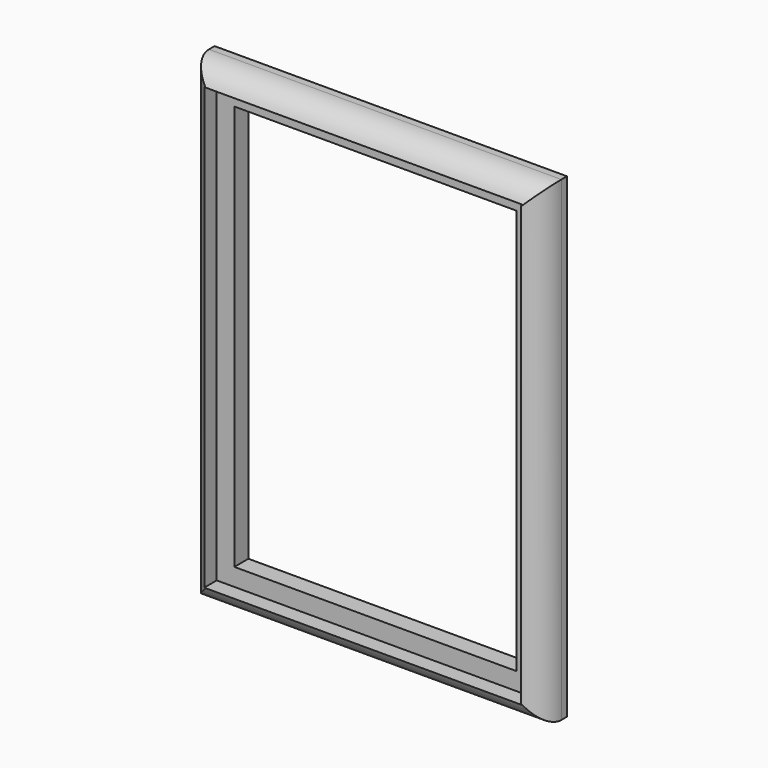
from build123d import *

# Parameters (mm, degrees)
F0_W        = 200
F0_H        = 270
F1_DEPTH    = 20
F2_W        = 180
F2_H        = 250
F3_DEPTH    = 10
F4_W        = 160
F4_H        = 230
F5_DEPTH    = 25
F6_T1_DEPTH = 350
F6_T3_DEPTH = 280


# Not quite as in the source:
# - a fillet or chamfer that OpenCascade refuses, or shapes differently, is made with other operations: its cross-section is extruded or revolved along the edge and cut away or added


with BuildPart() as f1:
    # F0 (on Front) → F1 (new body)
    with BuildSketch(Plane.XZ):
        with Locations((-21.7714021464, 1.2882190198)):
            Rectangle(F0_W, F0_H)
    extrude(amount=F1_DEPTH)

    # F2 (on face) → F3 (cut)
    with BuildSketch(Plane.XZ.offset(20)):
        with Locations((-22.5493634492, 1.4232655292)):
            Rectangle(F2_W, F2_H)
    extrude(amount=-F3_DEPTH, mode=Mode.SUBTRACT)

    # F4 (on face) → F5 (cut)
    with BuildSketch(Plane.XZ.offset(10)):
        with Locations((-22.5493634492, 1.4232655292)):
            Rectangle(F4_W, F4_H)
    extrude(amount=-F5_DEPTH, mode=Mode.SUBTRACT)

    # F6: fillet of radius 16 on 4 edges, made by hand

    # F6_s2 → F6_t1 (cut)
    with BuildSketch(Plane.XY.offset(-173.7117809802)):
        with BuildLine():
            ThreePointArc((-121.7714021464, -4), (-117.0851106454, -15.313708499), (-105.7714021464, -20))
            Line((-105.7714021464, -20), (-121.7714021464, -20))
            Line((-121.7714021464, -20), (-121.7714021464, -4))
        make_face()
        with BuildLine():
            ThreePointArc((62.2285978536, -20), (73.5423063526, -15.313708499), (78.2285978536, -4))
            Line((78.2285978536, -4), (78.2285978536, -20))
            Line((78.2285978536, -20), (62.2285978536, -20))
        make_face()
    extrude(amount=F6_T1_DEPTH, mode=Mode.SUBTRACT)

    # F6_s4 → F6_t3 (cut)
    with BuildSketch(Plane.YZ.offset(-161.7714021464)):
        with BuildLine():
            ThreePointArc((-4, 136.2882190198), (-15.313708499, 131.6019275188), (-20, 120.2882190198))
            Line((-20, 120.2882190198), (-20, 136.2882190198))
            Line((-20, 136.2882190198), (-4, 136.2882190198))
        make_face()
        with BuildLine():
            ThreePointArc((-4, -133.7117809802), (-15.313708499, -129.0254894792), (-20, -117.7117809802))
            Line((-20, -117.7117809802), (-20, -133.7117809802))
            Line((-20, -133.7117809802), (-4, -133.7117809802))
        make_face()
    extrude(amount=F6_T3_DEPTH, mode=Mode.SUBTRACT)


solid = f1.part
